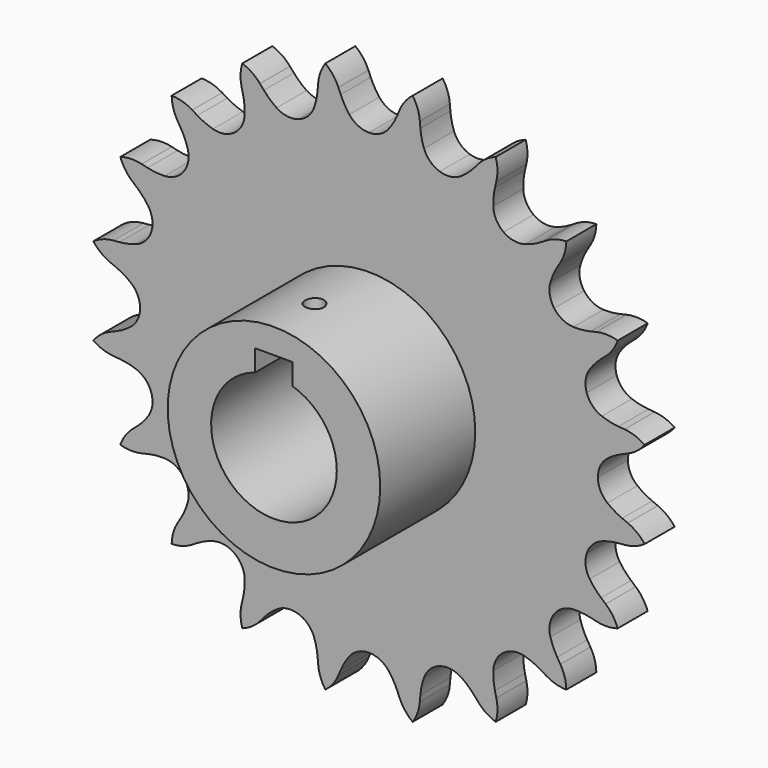
from build123d import *

# Parameters (mm, degrees)
F0_R     = 17
F1_DEPTH = 6
F2_DEPTH = 25
F3_R     = 1.5
F4_DEPTH = 25


# Not quite as in the source:
# - ends of sketch curves that miss each other by under 0.0002 mm in the source are joined


with BuildPart() as f1:
    # F0 (on Front) → F1 (new body)
    with BuildSketch(Plane.XZ):
        with BuildLine():
            ThreePointArc((0, 36.6108), (-1.7455398347, 37.0138545674), (-3.1376535005, 38.1414102602))
            ThreePointArc((-3.1376535005, 38.1414102602), (-3.9061352442, 39.2722549414), (-4.5183386939, 40.4947854399))
            Line((-4.5183386939, 40.4947854399), (-4.8877212466, 41.3735118089))
            Line((-4.8877212466, 41.3735118089), (-4.8994990247, 41.4015300358))
            ThreePointArc((-4.8994990247, 41.4015300358), (-5.7642620966, 42.881502078), (-6.9827152361, 44.0871288982))
            ThreePointArc((-6.9827152361, 44.0871288982), (-7.7689738578, 42.5639869277), (-8.1341464192, 40.8892293084))
            Line((-8.1341464192, 40.8892293084), (-8.1366191245, 40.8589369369))
            Line((-8.1366191245, 40.8589369369), (-8.2163814268, 39.9090730113))
            ThreePointArc((-8.2163814268, 39.9090730113), (-8.4208388068, 38.5571961444), (-8.8022581523, 37.2442250227))
            ThreePointArc((-8.8022581523, 37.2442250227), (-9.7778030544, 35.7416690528), (-11.3133593777, 34.8189399068))
            ThreePointArc((-11.3133593777, 34.8189399068), (-13.0980171229, 34.6628661063), (-14.7704297673, 35.3050485145))
            ThreePointArc((-14.7704297673, 35.3050485145), (-15.8507495619, 36.1430717988), (-16.8107723421, 37.1165861258))
            Line((-16.8107723421, 37.1165861258), (-17.4336174074, 37.8381590789))
            ThreePointArc((-17.4336174074, 37.8381590789), (-17.4435070012, 37.8496973523), (-17.4534232772, 37.8612127026))
            ThreePointArc((-17.4534232772, 37.8612127026), (-18.733251915, 39.0014770319), (-20.2646288894, 39.7715735486))
            ThreePointArc((-20.2646288894, 39.7715735486), (-20.5417285214, 38.0800121761), (-20.3714996997, 36.3743785018))
            Line((-20.3714996997, 36.3743785018), (-20.3644905245, 36.3448046365))
            Line((-20.3644905245, 36.3448046365), (-20.1468248866, 35.4167824536))
            ThreePointArc((-20.1468248866, 35.4167824536), (-19.9235224839, 34.067890345), (-19.8805434482, 32.7013155443))
            ThreePointArc((-19.8805434482, 32.7013155443), (-20.3440264546, 30.9708399445), (-21.5192883146, 29.6187593777))
            ThreePointArc((-21.5192883146, 29.6187593777), (-23.1683692359, 28.9188348003), (-24.9573734569, 29.0127826355))
            ThreePointArc((-24.9573734569, 29.0127826355), (-26.2437820737, 29.475952965), (-27.457650466, 30.1051567553))
            Line((-27.457650466, 30.1051567553), (-28.2729896291, 30.5989437043))
            ThreePointArc((-28.2729896291, 30.5989437043), (-28.2859607144, 30.6068612019), (-28.2989500922, 30.614748653))
            ThreePointArc((-28.2989500922, 30.614748653), (-29.8685005137, 31.3037156747), (-31.5628994752, 31.5628994752))
            ThreePointArc((-31.5628994752, 31.5628994752), (-31.3037156747, 29.8685005137), (-30.614748653, 28.2989500922))
            Line((-30.614748653, 28.2989500922), (-30.5989437043, 28.2729896291))
            Line((-30.5989437043, 28.2729896291), (-30.1051567553, 27.457650466))
            ThreePointArc((-30.1051567553, 27.457650466), (-29.475952965, 26.2437820737), (-29.0127826355, 24.9573734569))
            ThreePointArc((-29.0127826355, 24.9573734569), (-28.9188348003, 23.1683692359), (-29.6187593777, 21.5192883146))
            ThreePointArc((-29.6187593777, 21.5192883146), (-30.9708399445, 20.3440264546), (-32.7013155443, 19.8805434482))
            ThreePointArc((-32.7013155443, 19.8805434482), (-34.067890345, 19.9235224839), (-35.4167824536, 20.1468248866))
            Line((-35.4167824536, 20.1468248866), (-36.3448046365, 20.3644905245))
            ThreePointArc((-36.3448046365, 20.3644905245), (-36.3595875129, 20.3680122264), (-36.3743785018, 20.3714996997))
            ThreePointArc((-36.3743785018, 20.3714996997), (-38.0800121761, 20.5417285214), (-39.7715735486, 20.2646288894))
            ThreePointArc((-39.7715735486, 20.2646288894), (-39.0014770319, 18.733251915), (-37.8612127026, 17.4534232772))
            Line((-37.8612127026, 17.4534232772), (-37.8381590789, 17.4336174074))
            Line((-37.8381590789, 17.4336174074), (-37.1165861258, 16.8107723421))
            ThreePointArc((-37.1165861258, 16.8107723421), (-36.1430717988, 15.8507495619), (-35.3050485145, 14.7704297673))
            ThreePointArc((-35.3050485145, 14.7704297673), (-34.6628661063, 13.0980171229), (-34.8189399068, 11.3133593777))
            ThreePointArc((-34.8189399068, 11.3133593777), (-35.7416690528, 9.7778030544), (-37.2442250227, 8.8022581523))
            ThreePointArc((-37.2442250227, 8.8022581523), (-38.5571961444, 8.4208388068), (-39.9090730113, 8.2163814268))
            Line((-39.9090730113, 8.2163814268), (-40.8589369369, 8.1366191245))
            ThreePointArc((-40.8589369369, 8.1366191245), (-40.8740845536, 8.135400302), (-40.8892293084, 8.1341464192))
            ThreePointArc((-40.8892293084, 8.1341464192), (-42.5639869277, 7.7689738578), (-44.0871288982, 6.9827152361))
            ThreePointArc((-44.0871288982, 6.9827152361), (-42.881502078, 5.7642620966), (-41.4015574583, 4.8994337867))
            Line((-41.4015574583, 4.8994337867), (-41.3735118089, 4.8877212466))
            Line((-41.3735118089, 4.8877212466), (-40.4947854399, 4.5183386939))
            ThreePointArc((-40.4947854399, 4.5183386939), (-39.2722549414, 3.9061352442), (-38.1414102602, 3.1376535005))
            ThreePointArc((-38.1414102602, 3.1376535005), (-37.0138545674, 1.7455398347), (-36.6108, 0))
            ThreePointArc((-36.6108, 0), (-37.0138545674, -1.7455398347), (-38.1414102602, -3.1376535005))
            ThreePointArc((-38.1414102602, -3.1376535005), (-39.2722549414, -3.9061352442), (-40.4947854399, -4.5183386939))
            Line((-40.4947854399, -4.5183386939), (-41.3735118089, -4.8877212466))
            ThreePointArc((-41.3735118089, -4.8877212466), (-41.3875414116, -4.8935612867), (-41.4015574583, -4.8994337867))
            ThreePointArc((-41.4015574583, -4.8994337867), (-42.881502078, -5.7642620966), (-44.0871288982, -6.9827152361))
            ThreePointArc((-44.0871288982, -6.9827152361), (-42.5639869277, -7.7689738578), (-40.8892293084, -8.1341464192))
            Line((-40.8892293084, -8.1341464192), (-40.8589369369, -8.1366191245))
            Line((-40.8589369369, -8.1366191245), (-39.9090730113, -8.2163814268))
            ThreePointArc((-39.9090730113, -8.2163814268), (-38.5571961444, -8.4208388068), (-37.2442250227, -8.8022581523))
            ThreePointArc((-37.2442250227, -8.8022581523), (-35.7416690528, -9.7778030544), (-34.8189399068, -11.3133593777))
            ThreePointArc((-34.8189399068, -11.3133593777), (-34.6628661063, -13.0980171229), (-35.3050485145, -14.7704297673))
            ThreePointArc((-35.3050485145, -14.7704297673), (-36.1430717988, -15.8507495619), (-37.1165861258, -16.8107723421))
            Line((-37.1165861258, -16.8107723421), (-37.8381590789, -17.4336174074))
            ThreePointArc((-37.8381590789, -17.4336174074), (-37.8496973523, -17.4435070012), (-37.8612127026, -17.4534232772))
            ThreePointArc((-37.8612127026, -17.4534232772), (-39.0014770319, -18.733251915), (-39.7715735486, -20.2646288894))
            ThreePointArc((-39.7715735486, -20.2646288894), (-38.0800121761, -20.5417285214), (-36.3743785018, -20.3714996997))
            Line((-36.3743785018, -20.3714996997), (-36.3448046365, -20.3644905245))
            Line((-36.3448046365, -20.3644905245), (-35.4167824536, -20.1468248866))
            ThreePointArc((-35.4167824536, -20.1468248866), (-34.067890345, -19.9235224839), (-32.7013155443, -19.8805434482))
            ThreePointArc((-32.7013155443, -19.8805434482), (-30.9708399445, -20.3440264546), (-29.6187593777, -21.5192883146))
            ThreePointArc((-29.6187593777, -21.5192883146), (-28.9188348003, -23.1683692359), (-29.0127826355, -24.9573734569))
            ThreePointArc((-29.0127826355, -24.9573734569), (-29.475952965, -26.2437820737), (-30.1051567553, -27.457650466))
            Line((-30.1051567553, -27.457650466), (-30.5989437043, -28.2729896291))
            ThreePointArc((-30.5989437043, -28.2729896291), (-30.6068612019, -28.2859607144), (-30.614748653, -28.2989500922))
            ThreePointArc((-30.614748653, -28.2989500922), (-31.3037156747, -29.8685005137), (-31.5628994752, -31.5628994752))
            ThreePointArc((-31.5628994752, -31.5628994752), (-29.8685005137, -31.3037156747), (-28.2989500922, -30.614748653))
            Line((-28.2989500922, -30.614748653), (-28.2729896291, -30.5989437043))
            Line((-28.2729896291, -30.5989437043), (-27.457650466, -30.1051567553))
            ThreePointArc((-27.457650466, -30.1051567553), (-26.2437820737, -29.475952965), (-24.9573734569, -29.0127826355))
            ThreePointArc((-24.9573734569, -29.0127826355), (-23.1683692359, -28.9188348003), (-21.5192883146, -29.6187593777))
            ThreePointArc((-21.5192883146, -29.6187593777), (-20.3440264546, -30.9708399445), (-19.8805434482, -32.7013155443))
            ThreePointArc((-19.8805434482, -32.7013155443), (-19.9235224839, -34.067890345), (-20.1468248866, -35.4167824536))
            Line((-20.1468248866, -35.4167824536), (-20.3644905245, -36.3448046365))
            ThreePointArc((-20.3644905245, -36.3448046365), (-20.3680122264, -36.3595875129), (-20.3714996997, -36.3743785018))
            ThreePointArc((-20.3714996997, -36.3743785018), (-20.5417285214, -38.0800121761), (-20.2646288894, -39.7715735486))
            ThreePointArc((-20.2646288894, -39.7715735486), (-18.733251915, -39.0014770319), (-17.4534232772, -37.8612127026))
            Line((-17.4534232772, -37.8612127026), (-17.4336174074, -37.8381590789))
            Line((-17.4336174074, -37.8381590789), (-16.8107723421, -37.1165861258))
            ThreePointArc((-16.8107723421, -37.1165861258), (-15.8507495619, -36.1430717988), (-14.7704297673, -35.3050485145))
            ThreePointArc((-14.7704297673, -35.3050485145), (-13.0980171229, -34.6628661063), (-11.3133593777, -34.8189399068))
            ThreePointArc((-11.3133593777, -34.8189399068), (-9.7778030544, -35.7416690528), (-8.8022581523, -37.2442250227))
            ThreePointArc((-8.8022581523, -37.2442250227), (-8.4208388068, -38.5571961444), (-8.2163814268, -39.9090730113))
            Line((-8.2163814268, -39.9090730113), (-8.1366191245, -40.8589369369))
            ThreePointArc((-8.1366191245, -40.8589369369), (-8.135400302, -40.8740845536), (-8.1341464192, -40.8892293084))
            ThreePointArc((-8.1341464192, -40.8892293084), (-7.7689738578, -42.5639869277), (-6.9827152361, -44.0871288982))
            ThreePointArc((-6.9827152361, -44.0871288982), (-5.7642620966, -42.881502078), (-4.8994337867, -41.4015574583))
            Line((-4.8994337867, -41.4015574583), (-4.8877212466, -41.3735118089))
            Line((-4.8877212466, -41.3735118089), (-4.5183386939, -40.4947854399))
            ThreePointArc((-4.5183386939, -40.4947854399), (-3.9061352442, -39.2722549414), (-3.1376535005, -38.1414102602))
            ThreePointArc((-3.1376535005, -38.1414102602), (-1.7455398347, -37.0138545674), (0, -36.6108))
            ThreePointArc((0, -36.6108), (1.7455398347, -37.0138545674), (3.1376535005, -38.1414102602))
            ThreePointArc((3.1376535005, -38.1414102602), (3.9061352442, -39.2722549414), (4.5183386939, -40.4947854399))
            Line((4.5183386939, -40.4947854399), (4.8877212466, -41.3735118089))
            ThreePointArc((4.8877212466, -41.3735118089), (4.8935612867, -41.3875414116), (4.8994337867, -41.4015574583))
            ThreePointArc((4.8994337867, -41.4015574583), (5.7642620966, -42.881502078), (6.9827152361, -44.0871288982))
            ThreePointArc((6.9827152361, -44.0871288982), (7.7689738578, -42.5639869277), (8.1341464192, -40.8892293084))
            Line((8.1341464192, -40.8892293084), (8.1366191245, -40.8589369369))
            Line((8.1366191245, -40.8589369369), (8.2163814268, -39.9090730113))
            ThreePointArc((8.2163814268, -39.9090730113), (8.4208388068, -38.5571961444), (8.8022581523, -37.2442250227))
            ThreePointArc((8.8022581523, -37.2442250227), (9.7778030544, -35.7416690528), (11.3133593777, -34.8189399068))
            ThreePointArc((11.3133593777, -34.8189399068), (13.0980171229, -34.6628661063), (14.7704297673, -35.3050485145))
            ThreePointArc((14.7704297673, -35.3050485145), (15.8507495619, -36.1430717988), (16.8107723421, -37.1165861258))
            Line((16.8107723421, -37.1165861258), (17.4336174074, -37.8381590789))
            ThreePointArc((17.4336174074, -37.8381590789), (17.4435070012, -37.8496973523), (17.4534232772, -37.8612127026))
            ThreePointArc((17.4534232772, -37.8612127026), (18.733251915, -39.0014770319), (20.2646288894, -39.7715735486))
            ThreePointArc((20.2646288894, -39.7715735486), (20.5417285214, -38.0800121761), (20.3714996997, -36.3743785018))
            Line((20.3714996997, -36.3743785018), (20.3644905245, -36.3448046365))
            Line((20.3644905245, -36.3448046365), (20.1468248866, -35.4167824536))
            ThreePointArc((20.1468248866, -35.4167824536), (19.9235224839, -34.067890345), (19.8805434482, -32.7013155443))
            ThreePointArc((19.8805434482, -32.7013155443), (20.3440264546, -30.9708399445), (21.5192883146, -29.6187593777))
            ThreePointArc((21.5192883146, -29.6187593777), (23.1683692359, -28.9188348003), (24.9573734569, -29.0127826355))
            ThreePointArc((24.9573734569, -29.0127826355), (26.2437820737, -29.475952965), (27.457650466, -30.1051567553))
            Line((27.457650466, -30.1051567553), (28.2729896291, -30.5989437043))
            ThreePointArc((28.2729896291, -30.5989437043), (28.2859607144, -30.6068612019), (28.2989500922, -30.614748653))
            ThreePointArc((28.2989500922, -30.614748653), (29.8685005137, -31.3037156747), (31.5628994752, -31.5628994752))
            ThreePointArc((31.5628994752, -31.5628994752), (31.3037156747, -29.8685005137), (30.614748653, -28.2989500922))
            Line((30.614748653, -28.2989500922), (30.5989437043, -28.2729896291))
            Line((30.5989437043, -28.2729896291), (30.1051567553, -27.457650466))
            ThreePointArc((30.1051567553, -27.457650466), (29.475952965, -26.2437820737), (29.0127826355, -24.9573734569))
            ThreePointArc((29.0127826355, -24.9573734569), (28.9188348003, -23.1683692359), (29.6187593777, -21.5192883146))
            ThreePointArc((29.6187593777, -21.5192883146), (30.9708399445, -20.3440264546), (32.7013155443, -19.8805434482))
            ThreePointArc((32.7013155443, -19.8805434482), (34.067890345, -19.9235224839), (35.4167824536, -20.1468248866))
            Line((35.4167824536, -20.1468248866), (36.3448046365, -20.3644905245))
            ThreePointArc((36.3448046365, -20.3644905245), (36.3595875129, -20.3680122264), (36.3743785018, -20.3714996997))
            ThreePointArc((36.3743785018, -20.3714996997), (38.0800121761, -20.5417285214), (39.7715735486, -20.2646288894))
            ThreePointArc((39.7715735486, -20.2646288894), (39.0014770319, -18.733251915), (37.8612127026, -17.4534232772))
            Line((37.8612127026, -17.4534232772), (37.8381590789, -17.4336174074))
            Line((37.8381590789, -17.4336174074), (37.1165861258, -16.8107723421))
            ThreePointArc((37.1165861258, -16.8107723421), (36.1430717988, -15.8507495619), (35.3050485145, -14.7704297673))
            ThreePointArc((35.3050485145, -14.7704297673), (34.6628661063, -13.0980171229), (34.8189399068, -11.3133593777))
            ThreePointArc((34.8189399068, -11.3133593777), (35.7416690528, -9.7778030544), (37.2442250227, -8.8022581523))
            ThreePointArc((37.2442250227, -8.8022581523), (38.5571961444, -8.4208388068), (39.9090730113, -8.2163814268))
            Line((39.9090730113, -8.2163814268), (40.8589369369, -8.1366191245))
            ThreePointArc((40.8589369369, -8.1366191245), (40.8740845536, -8.135400302), (40.8892293084, -8.1341464192))
            ThreePointArc((40.8892293084, -8.1341464192), (42.5639869277, -7.7689738578), (44.0871288982, -6.9827152361))
            ThreePointArc((44.0871288982, -6.9827152361), (42.881502078, -5.7642620966), (41.4015574583, -4.8994337867))
            Line((41.4015574583, -4.8994337867), (41.3735118089, -4.8877212466))
            Line((41.3735118089, -4.8877212466), (40.4947854399, -4.5183386939))
            ThreePointArc((40.4947854399, -4.5183386939), (39.2722549414, -3.9061352442), (38.1414102602, -3.1376535005))
            ThreePointArc((38.1414102602, -3.1376535005), (37.0138545674, -1.7455398347), (36.6108, 0))
            ThreePointArc((36.6108, 0), (37.0138545674, 1.7455398347), (38.1414102602, 3.1376535005))
            ThreePointArc((38.1414102602, 3.1376535005), (39.2722549414, 3.9061352442), (40.4947854399, 4.5183386939))
            Line((40.4947854399, 4.5183386939), (41.3735118089, 4.8877212466))
            ThreePointArc((41.3735118089, 4.8877212466), (41.3875414116, 4.8935612867), (41.4015574583, 4.8994337867))
            ThreePointArc((41.4015574583, 4.8994337867), (42.881502078, 5.7642620966), (44.0871288982, 6.9827152361))
            ThreePointArc((44.0871288982, 6.9827152361), (42.5639869277, 7.7689738578), (40.8892293084, 8.1341464192))
            Line((40.8892293084, 8.1341464192), (40.8589369369, 8.1366191245))
            Line((40.8589369369, 8.1366191245), (39.9090730113, 8.2163814268))
            ThreePointArc((39.9090730113, 8.2163814268), (38.5571961444, 8.4208388068), (37.2442250227, 8.8022581523))
            ThreePointArc((37.2442250227, 8.8022581523), (35.7416690528, 9.7778030544), (34.8189399068, 11.3133593777))
            ThreePointArc((34.8189399068, 11.3133593777), (34.6628661063, 13.0980171229), (35.3050485145, 14.7704297673))
            ThreePointArc((35.3050485145, 14.7704297673), (36.1430717988, 15.8507495619), (37.1165861258, 16.8107723421))
            Line((37.1165861258, 16.8107723421), (37.8381590789, 17.4336174074))
            ThreePointArc((37.8381590789, 17.4336174074), (37.8496973523, 17.4435070012), (37.8612127026, 17.4534232772))
            ThreePointArc((37.8612127026, 17.4534232772), (39.0014770319, 18.733251915), (39.7715735486, 20.2646288894))
            ThreePointArc((39.7715735486, 20.2646288894), (38.0800121761, 20.5417285214), (36.3743785018, 20.3714996997))
            Line((36.3743785018, 20.3714996997), (36.3448046365, 20.3644905245))
            Line((36.3448046365, 20.3644905245), (35.4167824536, 20.1468248866))
            ThreePointArc((35.4167824536, 20.1468248866), (34.067890345, 19.9235224839), (32.7013155443, 19.8805434482))
            ThreePointArc((32.7013155443, 19.8805434482), (30.9708399445, 20.3440264546), (29.6187593777, 21.5192883146))
            ThreePointArc((29.6187593777, 21.5192883146), (28.9188348003, 23.1683692359), (29.0127826355, 24.9573734569))
            ThreePointArc((29.0127826355, 24.9573734569), (29.475952965, 26.2437820737), (30.1051567553, 27.457650466))
            Line((30.1051567553, 27.457650466), (30.5989437043, 28.2729896291))
            ThreePointArc((30.5989437043, 28.2729896291), (30.6068612019, 28.2859607144), (30.614748653, 28.2989500922))
            ThreePointArc((30.614748653, 28.2989500922), (31.3037156747, 29.8685005137), (31.5628994752, 31.5628994752))
            ThreePointArc((31.5628994752, 31.5628994752), (29.8685005137, 31.3037156747), (28.2989500922, 30.614748653))
            Line((28.2989500922, 30.614748653), (28.2729896291, 30.5989437043))
            Line((28.2729896291, 30.5989437043), (27.457650466, 30.1051567553))
            ThreePointArc((27.457650466, 30.1051567553), (26.2437820737, 29.475952965), (24.9573734569, 29.0127826355))
            ThreePointArc((24.9573734569, 29.0127826355), (23.1683692359, 28.9188348003), (21.5192883146, 29.6187593777))
            ThreePointArc((21.5192883146, 29.6187593777), (20.3440264546, 30.9708399445), (19.8805434482, 32.7013155443))
            ThreePointArc((19.8805434482, 32.7013155443), (19.9235224839, 34.067890345), (20.1468248866, 35.4167824536))
            Line((20.1468248866, 35.4167824536), (20.3644905245, 36.3448046365))
            ThreePointArc((20.3644905245, 36.3448046365), (20.3680122264, 36.3595875129), (20.3714996997, 36.3743785018))
            ThreePointArc((20.3714996997, 36.3743785018), (20.5417285214, 38.0800121761), (20.2646288894, 39.7715735486))
            ThreePointArc((20.2646288894, 39.7715735486), (18.733251915, 39.0014770319), (17.4534232772, 37.8612127026))
            Line((17.4534232772, 37.8612127026), (17.4336174074, 37.8381590789))
            Line((17.4336174074, 37.8381590789), (16.8107723421, 37.1165861258))
            ThreePointArc((16.8107723421, 37.1165861258), (15.8507495619, 36.1430717988), (14.7704297673, 35.3050485145))
            ThreePointArc((14.7704297673, 35.3050485145), (13.0980171229, 34.6628661063), (11.3133593777, 34.8189399068))
            ThreePointArc((11.3133593777, 34.8189399068), (9.7778030544, 35.7416690528), (8.8022581523, 37.2442250227))
            ThreePointArc((8.8022581523, 37.2442250227), (8.4208388068, 38.5571961444), (8.2163814268, 39.9090730113))
            Line((8.2163814268, 39.9090730113), (8.1366191245, 40.8589369369))
            ThreePointArc((8.1366191245, 40.8589369369), (8.135400302, 40.8740845536), (8.1341464192, 40.8892293084))
            ThreePointArc((8.1341464192, 40.8892293084), (7.7689738578, 42.5639869277), (6.9827152361, 44.0871288982))
            ThreePointArc((6.9827152361, 44.0871288982), (5.7642620966, 42.881502078), (4.8994337867, 41.4015574583))
            ThreePointArc((4.8994337867, 41.4015574583), (4.8935612867, 41.3875414116), (4.8877212466, 41.3735118089))
            Line((4.8877212466, 41.3735118089), (4.5183386939, 40.4947854399))
            ThreePointArc((4.5183386939, 40.4947854399), (3.9061352442, 39.2722549414), (3.1376535005, 38.1414102602))
            ThreePointArc((3.1376535005, 38.1414102602), (1.7455398347, 37.0138545674), (0, 36.6108))
        make_face()
        Circle(F0_R, mode=Mode.SUBTRACT)
        Circle(F0_R)
        with BuildLine():
            ThreePointArc((3, 9.5917933672), (8.0979163987, 5.9519954637), (10.05, 0))
            ThreePointArc((10.05, 0), (-5.9519954637, -8.0979163987), (-3, 9.5917933672))
            Line((-3, 9.5917933672), (-3, 13))
            Line((-3, 13), (3, 13))
            Line((3, 13), (3, 9.5917933672))
        make_face(mode=Mode.SUBTRACT)
    extrude(amount=F1_DEPTH)

    # F0 (on Front) → F2 (join)
    with BuildSketch(Plane.XZ):
        Circle(F0_R)
        with BuildLine():
            ThreePointArc((3, 9.5917933672), (8.0979163987, 5.9519954637), (10.05, 0))
            ThreePointArc((10.05, 0), (-5.9519954637, -8.0979163987), (-3, 9.5917933672))
            Line((-3, 9.5917933672), (-3, 13))
            Line((-3, 13), (3, 13))
            Line((3, 13), (3, 9.5917933672))
        make_face(mode=Mode.SUBTRACT)
    extrude(amount=F2_DEPTH)

    # F3 (on Top) → F4 (cut)
    with BuildSketch(Plane.XY):
        with Locations((0, -16.9105939567)):
            Circle(F3_R)
    extrude(amount=F4_DEPTH, mode=Mode.SUBTRACT)


solid = f1.part
